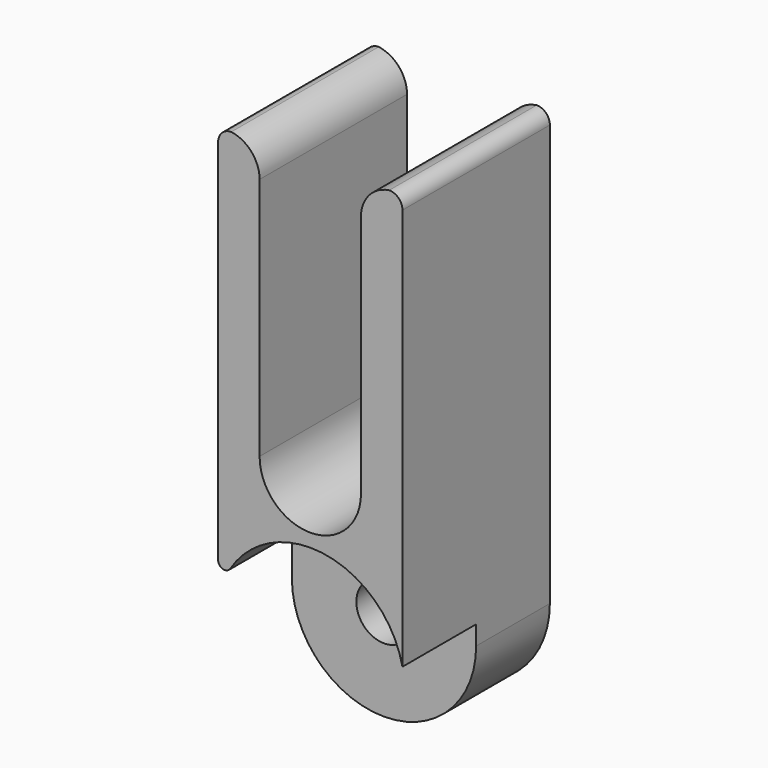
from build123d import *

# Parameters (mm, degrees)
F1_DEPTH    = 7
F2_R        = 1
F3_T1_DEPTH = 26.3768937945
F4_DEPTH    = 7
F5_D        = 4.2
F6_T1_DEPTH = 13.4425961547


# Not quite as in the source:
# - a fillet or chamfer that OpenCascade refuses, or shapes differently, is made with other operations: its cross-section is extruded or revolved along the edge and cut away or added


with BuildPart() as f1:
    # F0 (on Front) → F1 (new body, symmetric)
    with BuildSketch(Plane.XZ):
        with BuildLine():
            ThreePointArc((-7, 1.4568802284), (-4.5114191984, 5.5470349572), (0, 7.15))
            ThreePointArc((0, 7.15), (4.5114191984, 5.5470349572), (7, 1.4568802284))
            Line((7, 1.4568802284), (7, 33))
            Line((7, 33), (3.85, 33))
            Line((3.85, 33), (3.85, 12))
            ThreePointArc((3.85, 12), (2.7223611076, 9.2776388924), (0, 8.15))
            ThreePointArc((0, 8.15), (-2.7223611076, 9.2776388924), (-3.85, 12))
            Line((-3.85, 12), (-3.85, 33))
            Line((-3.85, 33), (-7, 33))
            Line((-7, 33), (-7, 1.4568802284))
        make_face()
    extrude(amount=F1_DEPTH, both=True)

    # F2
    f2_edges = [f1.edges().sort_by_distance(p)[0] for p in [
        (-7, 0, 33),
        (7, 0, 33),
    ]]
    fillet(f2_edges, radius=F2_R)

    # F3: fillet of radius 2.5 on 2 edges, made by hand

    # F3_s2 → F3_t1 (cut)
    with BuildSketch(Plane.XZ.offset(-13.1884468972)):
        with BuildLine():
            ThreePointArc((-6, 33), (-4.4625413912, 32.1639808722), (-3.85, 30.5246212411))
            Line((-3.85, 30.5246212411), (-3.8, 30.5246212411))
            Line((-3.8, 30.5246212411), (-3.8, 33))
            Line((-3.8, 33), (-3.85, 33.05))
            ThreePointArc((-3.85, 33.05), (-4.925, 33.05), (-5.993, 33.0495075752))
            Line((-5.993, 33.0495075752), (-6, 33))
        make_face()
        with BuildLine():
            ThreePointArc((6, 33), (4.4625413912, 32.1639808722), (3.85, 30.5246212411))
            Line((3.85, 30.5246212411), (3.8, 30.5246212411))
            Line((3.8, 30.5246212411), (3.8, 33))
            Line((3.8, 33), (3.85, 33.05))
            ThreePointArc((3.85, 33.05), (4.925, 33.05), (5.993, 33.0495075752))
            Line((5.993, 33.0495075752), (6, 33))
        make_face()
    extrude(amount=F3_T1_DEPTH, mode=Mode.SUBTRACT)

    # F0 (on Front) → F4 (join)
    with BuildSketch(Plane.XZ):
        with BuildLine():
            ThreePointArc((-7, 0), (-4.9497474683, 4.9497474683), (0, 7))
            Line((0, 7), (0, 7.15))
            ThreePointArc((0, 7.15), (-4.5114191984, 5.5470349572), (-7, 1.4568802284))
            Line((-7, 1.4568802284), (-7, 0))
        make_face()
        with BuildLine():
            Line((0, 7.15), (0, 7))
            ThreePointArc((0, 7), (4.9497474683, 4.9497474683), (7, 0))
            Line((7, 0), (7, 1.4568802284))
            ThreePointArc((7, 1.4568802284), (4.5114191984, 5.5470349572), (0, 7.15))
        make_face()
        with BuildLine():
            ThreePointArc((7, 0), (4.9497474683, 4.9497474683), (0, 7))
            Line((0, 7), (0, -7))
            ThreePointArc((0, -7), (4.9497474683, -4.9497474683), (7, 0))
        make_face()
        with BuildLine():
            Line((0, -7), (0, 7))
            ThreePointArc((0, 7), (-4.9497474683, 4.9497474683), (-7, 0))
            ThreePointArc((-7, 0), (-4.9497474683, -4.9497474683), (0, -7))
        make_face()
    extrude(amount=-F4_DEPTH)

    # F5 (through all)
    with Locations(Plane.XZ):
        with Locations((0, 0)):
            Hole(F5_D / 2)

    # F6: fillet of radius 0.5 on 1 edges, made by hand

    # F6_s2 → F6_t1 (cut)
    with BuildSketch(Plane.XZ):
        with BuildLine():
            ThreePointArc((-7, 4.0339186903), (-6.6370797201, 3.5530765641), (-6.0751633987, 3.7702638739))
            ThreePointArc((-6.0751633987, 3.7702638739), (-6.6391197043, 2.6541645675), (-7, 1.4568802284))
            Line((-7, 1.4568802284), (-7, 4.0339186903))
        make_face()
    extrude(amount=F6_T1_DEPTH, mode=Mode.SUBTRACT)


solid = f1.part
